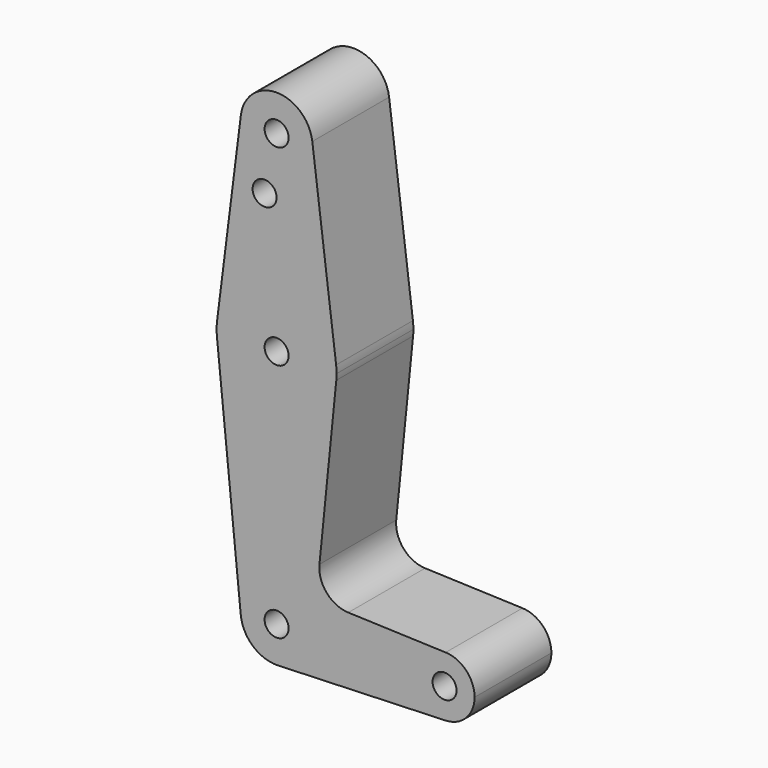
from build123d import *

# Parameters (mm, degrees)
F0_R     = 3.175
F1_DEPTH = 25.4


# Not quite as in the source:
# - a feature names something its author has since deleted; it is built from what else it names


with BuildPart() as f1:
    # F0 (on Front) → F1 (new body)
    with BuildSketch(Plane.XZ):
        with BuildLine():
            ThreePointArc((9.4502929642, 115.490625), (0, 123.825), (-9.4502929642, 115.490625))
            ThreePointArc((-9.4502929642, 115.490625), (-0.596483242, 104.7936951058), (9.525, 114.3))
            ThreePointArc((9.525, 114.3), (9.5063048942, 114.896483242), (9.4502929642, 115.490625))
        make_face()
        with Locations((0, 114.3)):
            Circle(F0_R, mode=Mode.SUBTRACT)
        with BuildLine():
            Line((-9.4502929642, 115.490625), (-15.7504882737, 65.484375))
            ThreePointArc((-15.7504882737, 65.484375), (0, 79.375), (15.7504882737, 65.484375))
            Line((15.7504882737, 65.484375), (9.4502929642, 115.490625))
            ThreePointArc((9.4502929642, 115.490625), (9.5063048942, 114.896483242), (9.525, 114.3))
            ThreePointArc((9.525, 114.3), (-0.596483242, 104.7936951058), (-9.4502929642, 115.490625))
        make_face()
        with Locations((-3.175, 99.3271544576)):
            Circle(F0_R, mode=Mode.SUBTRACT)
        with BuildLine():
            ThreePointArc((-15.7504882737, 65.484375), (-15.8737438155, 63.6997054867), (-15.7954255641, 61.9125))
            ThreePointArc((-15.7954255641, 61.9125), (0, 47.625), (15.7954255641, 61.9125))
            ThreePointArc((15.7954255641, 61.9125), (15.8550939106, 62.7052534459), (15.875, 63.5))
            ThreePointArc((15.875, 63.5), (15.8438414904, 64.4941387366), (15.7504882737, 65.484375))
            ThreePointArc((15.7504882737, 65.484375), (0, 79.375), (-15.7504882737, 65.484375))
        make_face()
        with Locations((0, 63.5)):
            Circle(F0_R, mode=Mode.SUBTRACT)
        with BuildLine():
            ThreePointArc((-9.4772553384, -0.9525), (-0.4768479324, 9.5130563464), (9.525, 0))
            Line((9.525, 0), (36.5125, 0))
            ThreePointArc((36.5125, 0), (38.9384772185, 5.7120069047), (44.7334821429, 7.9324362036))
            Line((44.7334821429, 7.9324362036), (18.9676000005, 8.8532337108))
            ThreePointArc((18.9676000005, 8.8532337108), (13.2611998974, 11.5713591498), (11.3411865923, 17.5933818124))
            Line((11.3411865923, 17.5933818124), (15.7954255641, 61.9125))
            ThreePointArc((15.7954255641, 61.9125), (0, 47.625), (-15.7954255641, 61.9125))
            Line((-15.7954255641, 61.9125), (-9.4772553384, -0.9525))
        make_face()
        with BuildLine():
            ThreePointArc((0.3401785714, -9.5189234444), (6.8544082857, -6.6138273378), (9.525, 0))
            ThreePointArc((9.525, 0), (-0.4768479324, 9.5130563464), (-9.4772553384, -0.9525))
            ThreePointArc((-9.4772553384, -0.9525), (-6.2623833816, -7.1769199091), (0.3401785714, -9.5189234444))
        make_face()
        Circle(F0_R, mode=Mode.SUBTRACT)
        with BuildLine():
            Line((36.5125, 0), (9.525, 0))
            ThreePointArc((9.525, 0), (6.8544082857, -6.6138273378), (0.3401785714, -9.5189234444))
            Line((0.3401785714, -9.5189234444), (44.7334821429, -7.9324362036))
            ThreePointArc((44.7334821429, -7.9324362036), (38.9384772185, -5.7120069047), (36.5125, 0))
        make_face()
        with BuildLine():
            ThreePointArc((44.7334821429, 7.9324362036), (38.9384772185, 5.7120069047), (36.5125, 0))
            ThreePointArc((36.5125, 0), (38.9384772185, -5.7120069047), (44.7334821429, -7.9324362036))
            ThreePointArc((44.7334821429, -7.9324362036), (50.1620069047, -5.5115227815), (52.3875, 0))
            ThreePointArc((52.3875, 0), (50.1620069047, 5.5115227815), (44.7334821429, 7.9324362036))
        make_face()
        with BuildLine():
            ThreePointArc((47.625, 0), (44.45, -3.175), (41.275, 0))
            ThreePointArc((41.275, 0), (44.45, 3.175), (47.625, 0))
        make_face(mode=Mode.SUBTRACT)
    extrude(amount=F1_DEPTH)


solid = f1.part
